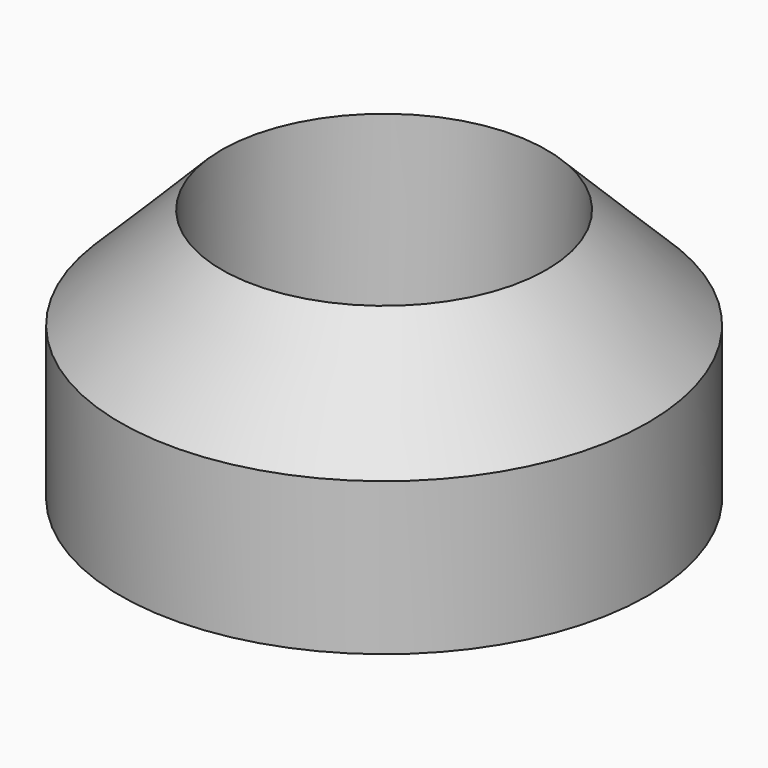
from build123d import *

# Parameters (mm, degrees)
F0_R     = 5.2
F0_R_2   = 3.2
F1_DEPTH = 5
F2_SIZE  = 1.99999


# Not quite as in the source:
# - a fillet or chamfer is up to 0.001 mm smaller than in the source, because OpenCascade refuses the exact size


with BuildPart() as f1:
    # F0 (on Top) → F1 (new body)
    with BuildSketch(Plane.XY):
        Circle(F0_R)
        Circle(F0_R_2, mode=Mode.SUBTRACT)
    extrude(amount=F1_DEPTH)

    # F2 (size 2 in the source; OpenCascade refuses exactly that, so slightly less here)
    f2_edges = [f1.edges().sort_by_distance(p)[0] for p in [
        (-5.2, 0, 5),
    ]]
    chamfer(f2_edges, length=F2_SIZE)


solid = f1.part
